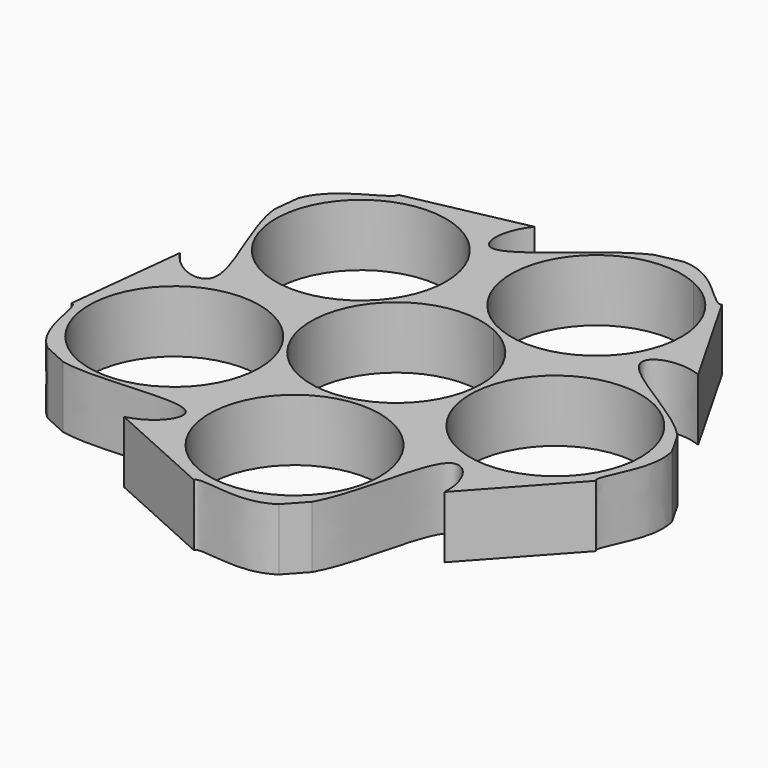
from build123d import *

# Parameters (mm, degrees)
F1_DEPTH        = 8
F3_DEPTH        = 7.62
F2_R            = 11
F4_DEPTH        = 8.001
F6_DEPTH        = 8.001
F6_COPIES_COUNT = 5


# Not quite as in the source:
# - a pattern or mirror of a feature is missing from the dataset's text; its kind, count and spacing are read off the source's solid


with BuildPart() as f1:
    # F0 (on Top) → F1 (new body)
    with BuildSketch(Plane.XY):
        Polygon((-28.197217237, 25.6227816618), (-33.0821327854, -18.899272218), (7.7513347553, -37.3031742552), (37.8727211223, -4.1553573599), (15.6552941447, 34.7350221713), align=None)
    extrude(amount=F1_DEPTH)

    # F0 (on Top) → F3 (join)
    with BuildSketch(Plane.XY):
        Polygon((-28.197217237, 25.6227816618), (-33.0821327854, -18.899272218), (7.7513347553, -37.3031742552), (37.8727211223, -4.1553573599), (15.6552941447, 34.7350221713), align=None)
    extrude(amount=F3_DEPTH)

    # F2 (on face) → F4 (cut, through all)
    with BuildSketch(Plane.XY.offset(8)):
        with BuildLine():
            ThreePointArc((4.7915254271, 10.6311475469), (15.2813967592, 11.4206134773), (20.3114266237, 20.6596316384))
            ThreePointArc((20.3114266237, 20.6596316384), (18.5504447848, 26.6296017738), (13.8313278203, 30.6881157298))
            Line((13.8313278203, 30.6881157298), (4.7915254271, 10.6311475469))
        make_face()
        with BuildLine():
            ThreePointArc((11, 0), (9.2390181611, 5.9699701355), (4.5199011966, 10.0284840915))
            Line((4.5199011966, 10.0284840915), (-4.5199011966, -10.0284840915))
            ThreePointArc((-4.5199011966, -10.0284840915), (5.9699701355, -9.2390181611), (11, 0))
        make_face()
        with BuildLine():
            Line((-4.5199011966, -10.0284840915), (4.5199011966, 10.0284840915))
            ThreePointArc((4.5199011966, 10.0284840915), (-10.0284840915, 4.5199011966), (-4.5199011966, -10.0284840915))
        make_face()
        with BuildLine():
            Line((4.7915254271, 10.6311475469), (13.8313278203, 30.6881157298))
            ThreePointArc((13.8313278203, 30.6881157298), (-0.7170574678, 25.179532835), (4.7915254271, 10.6311475469))
        make_face()
        with Locations((-16.7710882253, 15.2398702403)):
            Circle(F2_R)
        with Locations((-19.6765291753, -11.2408738458)):
            Circle(F2_R)
        with Locations((4.6103244144, -22.1871123402)):
            Circle(F2_R)
        with Locations((22.5258663625, -2.4715156927)):
            Circle(F2_R)
    extrude(amount=-F4_DEPTH, mode=Mode.SUBTRACT)

    # F5 (on face) → F6 (cut, through all)
    with BuildSketch(Plane.XY.offset(8)):
        with BuildLine():
            add(Edge.make_bspline(
                [(22.8120279388, -20.7292658076), (23.002965141, -17.2683955118), (17.6285578787, -10.4206910475), (15.7845912852, -33.2454047485), (6.8246182254, -35.0204881907), (-1.1481771733, -33.2421265212), (9.5130243684, -41.9931634056), (22.452896828, -27.2387683029), (22.8120279388, -20.7292658076)],
                knots=[0, 0, 0, 0, 0.1324484051, 0.3459771616, 0.5004726067, 0.6122390719, 0.7508796488, 1, 1, 1, 1], degree=3))
        make_face()
    f6 = extrude(amount=-F6_DEPTH, mode=Mode.SUBTRACT)

    # F6_copies: F6 ×5 about axis
    f6_copies_axis = Axis((0, 0, 0), (0, 0, 1))
    for i in range(1, F6_COPIES_COUNT):
        add(f6.rotate(f6_copies_axis, i * 360 / F6_COPIES_COUNT), mode=Mode.SUBTRACT)


solid = f1.part
